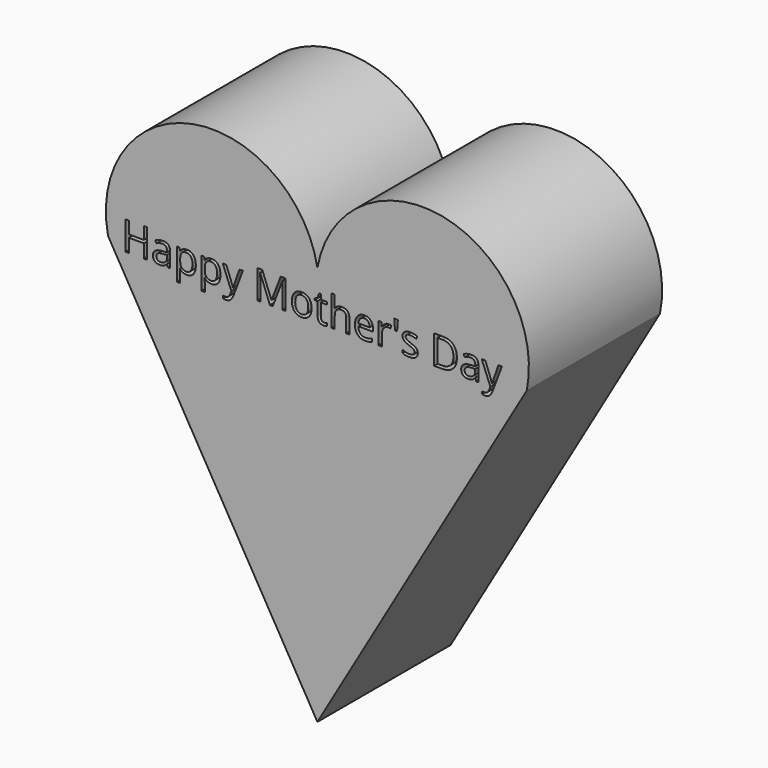
from build123d import *

# Parameters (mm, degrees)
F1_DEPTH     = 25.4
F2_TEXT_SIZE = 6.1253952391
F3_DEPTH     = 12.7


# Not quite as in the source:
# - Text() gives the source's letters only with a copy of the font that has no kerning and outlines rounded to 1/6400 em; it was checked with that copy


with BuildPart() as f1:
    # F0 (on Front) → F1 (new body)
    with BuildSketch(Plane.XZ):
        with BuildLine():
            Line((0, 21.8297690153), (0, -33.466224515))
            Line((0, -33.466224515), (31.9363405297, 21.4183831048))
            ThreePointArc((31.9363405297, 21.4183831048), (19.0458543535, 40.6318655113), (0, 27.4949719671))
            ThreePointArc((0, 27.4949719671), (0.2486921414, 24.6623704912), (0, 21.8297690153))
        make_face()
        with BuildLine():
            Line((-31.9363405297, 21.4183831048), (0, -33.466224515))
            Line((0, -33.466224515), (0, 21.8297690153))
            ThreePointArc((0, 21.8297690153), (-0.2486921414, 24.6623704912), (0, 27.4949719671))
            ThreePointArc((0, 27.4949719671), (-19.0458543535, 40.6318655113), (-31.9363405297, 21.4183831048))
        make_face()
        with BuildLine():
            ThreePointArc((0, 27.4949719671), (-0.2486921414, 24.6623704912), (0, 21.8297690153))
            ThreePointArc((0, 21.8297690153), (0.2486921414, 24.6623704912), (0, 27.4949719671))
        make_face()
    extrude(amount=F1_DEPTH)

    # F2 (on face) → F3 (cut)
    with BuildSketch(Plane.XZ.offset(25.4)):
        with Locations((-29.8808125064, 20.1400169886)):
            Text("Happy Mother's Day", F2_TEXT_SIZE, font='Open Sans', text_align=(TextAlign.LEFT, TextAlign.BOTTOM))
    extrude(amount=-F3_DEPTH, mode=Mode.SUBTRACT)


solid = f1.part
